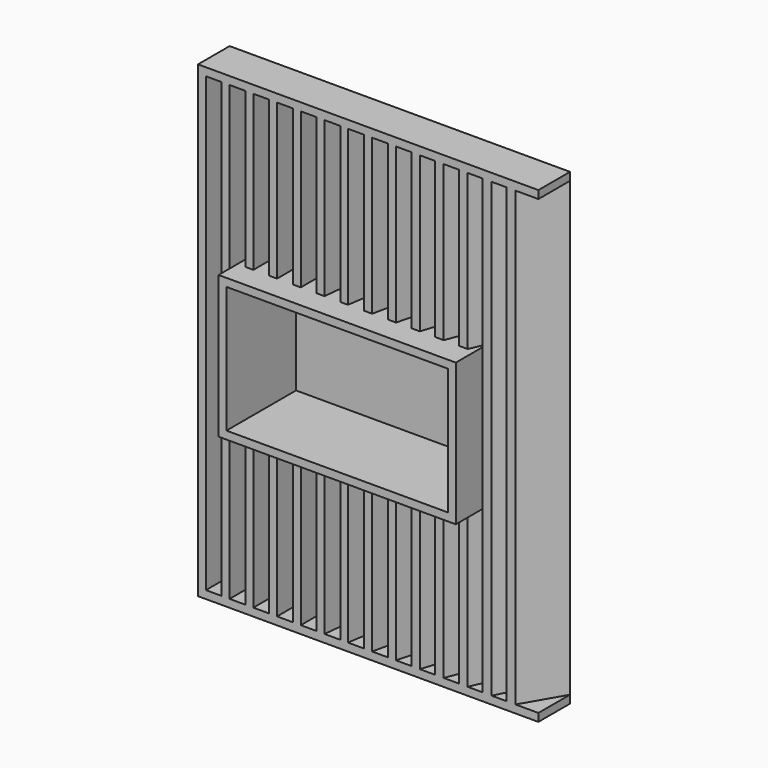
from build123d import *

# Parameters (mm, degrees)
F0_W          = 50
F0_H          = 250
F1_DEPTH      = 2860
F2_W          = 2221.6949462891
F2_H          = 250
F3_DEPTH      = 2860.001
F5_W          = 2152.0382275355
F5_H          = 250
F6_DEPTH      = 50
F7_W          = 1500
F7_H          = 900
F8_DEPTH      = 150
F8_DEPTH_BACK = 450
F10_W         = 1400
F10_H         = 800
F11_DEPTH     = 550


# Not quite as in the source:
# - a pattern or mirror of a feature is missing from the dataset's text; its kind, count and spacing are read off the source's solid


with BuildPart() as f1:
    # F0 (on Top) → F1 (new body)
    with BuildSketch(Plane.XY):
        with Locations((25, 125)):
            Rectangle(F0_W, F0_H)
    extrude(amount=F1_DEPTH)


with BuildPart() as f1b:
    # F0 (on Top) → F1, piece 2 (new body)
    with BuildSketch(Plane.XY):
        with Locations((175, 125)):
            Rectangle(F0_W, F0_H)
    extrude(amount=F1_DEPTH)


with BuildPart() as f1c:
    # F0 (on Top) → F1, piece 3 (new body)
    with BuildSketch(Plane.XY):
        with Locations((325, 125)):
            Rectangle(F0_W, F0_H)
    extrude(amount=F1_DEPTH)


with BuildPart() as f1d:
    # F0 (on Top) → F1, piece 4 (new body)
    with BuildSketch(Plane.XY):
        with Locations((475, 125)):
            Rectangle(F0_W, F0_H)
    extrude(amount=F1_DEPTH)


with BuildPart() as f1e:
    # F0 (on Top) → F1, piece 5 (new body)
    with BuildSketch(Plane.XY):
        with Locations((625, 125)):
            Rectangle(F0_W, F0_H)
    extrude(amount=F1_DEPTH)


with BuildPart() as f1f:
    # F0 (on Top) → F1, piece 6 (new body)
    with BuildSketch(Plane.XY):
        Polygon((776.5894605545, 255.2512190888), (750, 0), (799.7260947684, -5.2264231634), (826.5514727946, 250), align=None)
    extrude(amount=F1_DEPTH)


with BuildPart() as f1g:
    # F0 (on Top) → F1, piece 7 (new body)
    with BuildSketch(Plane.XY):
        Polygon((1985.7988202348, 254.516253274), (1932.2269349213, 259.5099715872), (1800, 0), (1844.5503262094, -22.699524987), align=None)
    extrude(amount=F1_DEPTH)


with BuildPart() as f1h:
    # F0 (on Top) → F1, piece 8 (new body)
    with BuildSketch(Plane.XY):
        Polygon((2220.7730672405, 369.0522346192), (2179.9817015181, 392.6031405997), (1950, 0), (1994.1379562017, -23.491292479), align=None)
    extrude(amount=F1_DEPTH)


with BuildPart() as f1i:
    # F0 (on Top) → F1, piece 9 (new body)
    with BuildSketch(Plane.XY):
        Polygon((954.1632750594, 341.9734599461), (900, 0), (944.2202974276, -23.3359228533), (1000.9070231543, 334.5699775654), align=None)
    extrude(amount=F1_DEPTH)


with BuildPart() as f1j:
    # F0 (on Top) → F1, piece 10 (new body)
    with BuildSketch(Plane.XY):
        Polygon((1122.346880499, 340.3653123223), (1050, 0), (1098.9073800367, -10.3955845409), (1171.2542605357, 329.9697277814), align=None)
    extrude(amount=F1_DEPTH)


with BuildPart() as f1k:
    # F0 (on Top) → F1, piece 11 (new body)
    with BuildSketch(Plane.XY):
        Polygon((1287.782294212, 327.6079820043), (1200, 0), (1247.5893550212, -15.3379688571), (1336.018259136, 314.6831941568), align=None)
    extrude(amount=F1_DEPTH)


with BuildPart() as f1l:
    # F0 (on Top) → F1, piece 12 (new body)
    with BuildSketch(Plane.XY):
        Polygon((1436.4378824264, 266.0284477321), (1350, 0), (1397.5528258148, -15.4508497187), (1483.8030352701, 250), align=None)
    extrude(amount=F1_DEPTH)


with BuildPart() as f1m:
    # F0 (on Top) → F1, piece 13 (new body)
    with BuildSketch(Plane.XY):
        Polygon((1601.4181799658, 264.2033915901), (1500, 0), (1546.6790213249, -17.9183974773), (1650.8878155953, 253.5547929215), align=None)
    extrude(amount=F1_DEPTH)


with BuildPart() as f1n:
    # F0 (on Top) → F1, piece 14 (new body)
    with BuildSketch(Plane.XY):
        Polygon((1775.6190094628, 282.1449147549), (1650, 0), (1697.1604126952, -16.6101015777), (1821.1493091009, 261.8735193053), align=None)
    extrude(amount=F1_DEPTH)


with BuildPart() as f3_tool:
    # F2 (on Top) → F3 (new body, through all)
    with BuildSketch(Plane.XY):
        with Locations((1110.8474731445, 125)):
            Rectangle(F2_W, F2_H)
    extrude(amount=F3_DEPTH)


with BuildPart() as f1_1:
    add(f1.part)

    # F3: intersect by f3_tool
    add(f3_tool.part, mode=Mode.INTERSECT)



with BuildPart() as f1b_1:
    add(f1b.part)

    # F3: intersect by f3_tool
    add(f3_tool.part, mode=Mode.INTERSECT)


with BuildPart() as f1c_1:
    add(f1c.part)

    # F3: intersect by f3_tool
    add(f3_tool.part, mode=Mode.INTERSECT)


with BuildPart() as f1d_1:
    add(f1d.part)

    # F3: intersect by f3_tool
    add(f3_tool.part, mode=Mode.INTERSECT)


with BuildPart() as f1e_1:
    add(f1e.part)

    # F3: intersect by f3_tool
    add(f3_tool.part, mode=Mode.INTERSECT)


with BuildPart() as f1f_1:
    add(f1f.part)

    # F3: intersect by f3_tool
    add(f3_tool.part, mode=Mode.INTERSECT)


with BuildPart() as f1g_1:
    add(f1g.part)

    # F3: intersect by f3_tool
    add(f3_tool.part, mode=Mode.INTERSECT)


with BuildPart() as f1h_1:
    add(f1h.part)

    # F3: intersect by f3_tool
    add(f3_tool.part, mode=Mode.INTERSECT)


with BuildPart() as f1i_1:
    add(f1i.part)

    # F3: intersect by f3_tool
    add(f3_tool.part, mode=Mode.INTERSECT)


with BuildPart() as f1j_1:
    add(f1j.part)

    # F3: intersect by f3_tool
    add(f3_tool.part, mode=Mode.INTERSECT)


with BuildPart() as f1k_1:
    add(f1k.part)

    # F3: intersect by f3_tool
    add(f3_tool.part, mode=Mode.INTERSECT)


with BuildPart() as f1l_1:
    add(f1l.part)

    # F3: intersect by f3_tool
    add(f3_tool.part, mode=Mode.INTERSECT)


with BuildPart() as f1m_1:
    add(f1m.part)

    # F3: intersect by f3_tool
    add(f3_tool.part, mode=Mode.INTERSECT)


with BuildPart() as f1n_1:
    add(f1n.part)

    # F3: intersect by f3_tool
    add(f3_tool.part, mode=Mode.INTERSECT)


with BuildPart() as f1_2:
    add(f1_1.part)

    add(f1b_1.part)  # F6 merges F1b

    add(f1c_1.part)  # F6 merges F1c

    add(f1d_1.part)  # F6 merges F1d

    add(f1e_1.part)  # F6 merges F1e

    add(f1f_1.part)  # F6 merges F1f

    add(f1g_1.part)  # F6 merges F1g

    add(f1h_1.part)  # F6 merges F1h

    add(f1i_1.part)  # F6 merges F1i

    add(f1j_1.part)  # F6 merges F1j

    add(f1k_1.part)  # F6 merges F1k

    add(f1l_1.part)  # F6 merges F1l

    add(f1m_1.part)  # F6 merges F1m

    add(f1n_1.part)  # F6 merges F1n
    # F5 (on Top) → F6 (join)
    with BuildSketch(Plane.XY):
        with Locations((1076.0191137678, 125)):
            Rectangle(F5_W, F5_H)
    f6 = extrude(amount=-F6_DEPTH)

    # F6_copies: F6 across plane
    add(f6.mirror(Plane.XY.offset(1430)))


with BuildPart() as f8:
    # F7 (on Front) → F8 (new body, two sides)
    with BuildSketch(Plane.XZ) as f8_sk:
        with Locations((1000, 1430)):
            Rectangle(F7_W, F7_H)
    extrude(amount=F8_DEPTH)
    extrude(f8_sk.sketch, amount=-F8_DEPTH_BACK)


with BuildPart() as f1_3:
    add(f1_2.part)

    # F9: cut F8
    add(f8.part, mode=Mode.SUBTRACT)


with BuildPart() as f8_1:
    add(f8.part)

    # F10 (on face) → F11 (cut)
    with BuildSketch(Plane.XZ.offset(150)):
        with Locations((1000, 1430)):
            Rectangle(F10_W, F10_H)
    extrude(amount=-F11_DEPTH, mode=Mode.SUBTRACT)


solid = Compound([f1_3.part, f8_1.part])
